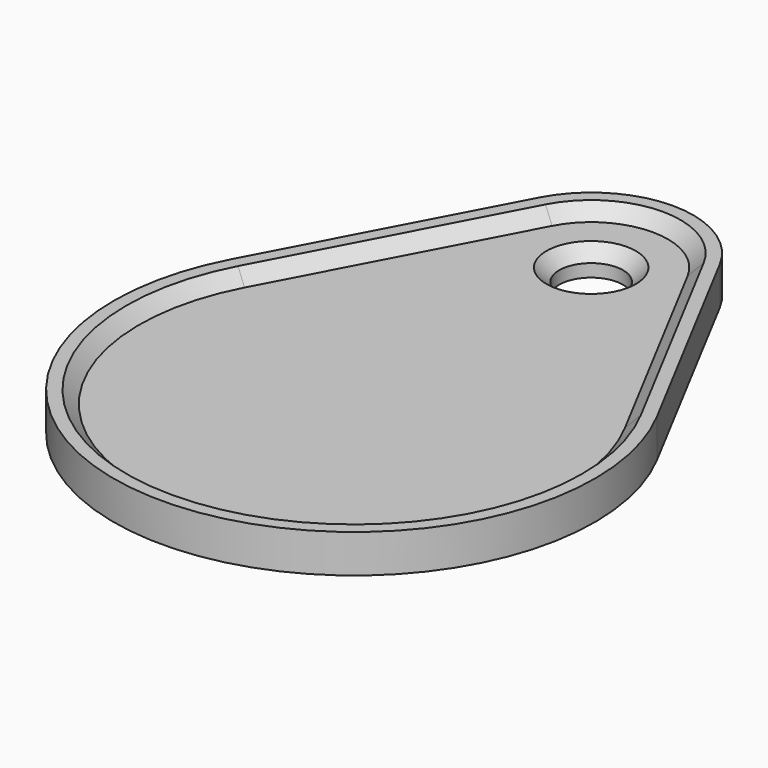
from build123d import *

# Parameters (mm, degrees)
F1_DEPTH = 3
F2_R     = 2.5
F3_DEPTH = 25
F5_DEPTH = 1
F6_SIZE  = 0.99999


# Not quite as in the source:
# - a fillet or chamfer is up to 0.001 mm smaller than in the source, because OpenCascade refuses the exact size


with BuildPart() as f1:
    # F0 (on Top) → F1 (new body)
    with BuildSketch(Plane.XY):
        with BuildLine():
            Line((-7.0720659795, 18.1059757224), (-16.646664491, 0))
            ThreePointArc((-16.646664491, 0), (0, -27.6337946959), (16.646664491, 0))
            Line((16.646664491, 0), (7.0720659795, 18.1059757224))
            ThreePointArc((7.0720659795, 18.1059757224), (0, 22.3662053041), (-7.0720659795, 18.1059757224))
        make_face()
    extrude(amount=F1_DEPTH)

    # F2 (on face) → F3 (cut)
    with BuildSketch(Plane.XY.offset(3)):
        with Locations((0, 14.3662053041)):
            Circle(F2_R)
    extrude(amount=-F3_DEPTH, mode=Mode.SUBTRACT)

    # F4 (on face) → F5 (cut)
    with BuildSketch(Plane.XY.offset(3)):
        with BuildLine():
            Line((15.7626562435, -0.4674713023), (6.1880577321, 17.6385044201))
            ThreePointArc((6.1880577321, 17.6385044201), (0, 21.3662053041), (-6.1880577321, 17.6385044201))
            Line((-6.1880577321, 17.6385044201), (-15.7626562435, -0.4674713023))
            ThreePointArc((-15.7626562435, -0.4674713023), (0, -26.6337946959), (15.7626562435, -0.4674713023))
        make_face()
    extrude(amount=-F5_DEPTH, mode=Mode.SUBTRACT)

    # F6 (size 1 in the source; OpenCascade refuses exactly that, so slightly less here)
    f6_edges = [f1.edges().sort_by_distance(p)[0] for p in [
        (0, -26.633795, 2),
        (-10.975357, 8.585517, 2),
        (10.975357, 8.585517, 2),
        (0, 21.366205, 2),
        (-2.5, 14.366205, 2),
    ]]
    chamfer(f6_edges, length=F6_SIZE)


solid = f1.part
